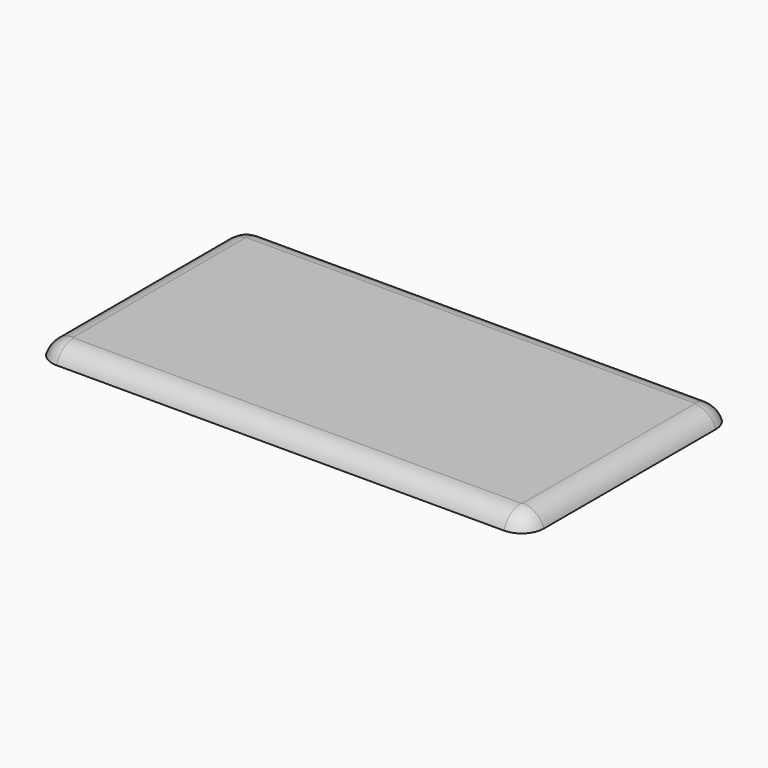
from build123d import *

# Parameters (mm, degrees)
F1_DEPTH     = 3.5
F5_D         = 4.473
F5_DEPTH     = 0.8
F5_TIP       = 1.3438247745
F6_T1_DEPTH  = 101
F6_T3_DEPTH  = 48.5
F6_T6_ANGLE  = 90
F6_T8_ANGLE  = 90
F6_T10_ANGLE = 90
F6_T12_ANGLE = 90
F8_W         = 0.5
F8_H         = 37.5
F8_W_2       = 88
F8_H_2       = 0.5
F9_DEPTH     = 1


# Not quite as in the source:
# - a fillet or chamfer that OpenCascade refuses, or shapes differently, is made with other operations: its cross-section is extruded or revolved along the edge and cut away or added


with BuildPart() as f1:
    # F0 (on Top) → F1 (new body)
    with BuildSketch(Plane.XY):
        with BuildLine():
            Line((-50.5, -29.25), (50.5, -29.25))
            ThreePointArc((50.5, -29.25), (54.0355339059, -27.7855339059), (55.5, -24.25))
            Line((55.5, -24.25), (55.5, 24.25))
            ThreePointArc((55.5, 24.25), (54.0355339059, 27.7855339059), (50.5, 29.25))
            Line((50.5, 29.25), (-50.5, 29.25))
            ThreePointArc((-50.5, 29.25), (-54.0355339059, 27.7855339059), (-55.5, 24.25))
            Line((-55.5, 24.25), (-55.5, -24.25))
            ThreePointArc((-55.5, -24.25), (-54.0355339059, -27.7855339059), (-50.5, -29.25))
        make_face()
    extrude(amount=F1_DEPTH)

    # F5
    with Locations(Plane(origin=(0, 0, 0), x_dir=(1, 0, 0), z_dir=(0, 0, -1))):
        with Locations((-50.2406740561, -23.9985361695), (-50.2495961264, 24.0030474961), (50.2488752827, 23.995583877), (50.2413948998, -24.0000952035)):
            Hole(F5_D / 2, depth=F5_DEPTH)
            with Locations((0, 0, -(F5_DEPTH + F5_TIP / 2))):  # 118° drill point
                Cone(0, F5_D / 2, F5_TIP, mode=Mode.SUBTRACT)

    # F6: fillet of radius 5 on 1 edges, made by hand

    # F6_s2 → F6_t1 (cut)
    with BuildSketch(Plane.YZ.offset(-50.5)):
        with BuildLine():
            ThreePointArc((-29.25, 0), (-27.4383438845, 2.5311288741), (-24.4803039929, 3.5))
            Line((-24.4803039929, 3.5), (-29.25, 3.5))
            Line((-29.25, 3.5), (-29.25, 0))
        make_face()
        with BuildLine():
            ThreePointArc((24.4803039929, 3.5), (27.4383438845, 2.5311288741), (29.25, 0))
            Line((29.25, 0), (29.25, 3.5))
            Line((29.25, 3.5), (24.4803039929, 3.5))
        make_face()
    extrude(amount=F6_T1_DEPTH, mode=Mode.SUBTRACT)

    # F6_s4 → F6_t3 (cut)
    with BuildSketch(Plane.XZ.offset(-24.25)):
        with BuildLine():
            ThreePointArc((50.7303039929, 3.5), (53.6883438845, 2.5311288741), (55.5, 0))
            Line((55.5, 0), (55.5, 3.5))
            Line((55.5, 3.5), (50.7303039929, 3.5))
        make_face()
        with BuildLine():
            ThreePointArc((-50.7303039929, 3.5), (-53.6883438845, 2.5311288741), (-55.5, 0))
            Line((-55.5, 0), (-55.5, 3.5))
            Line((-55.5, 3.5), (-50.7303039929, 3.5))
        make_face()
    extrude(amount=F6_T3_DEPTH, mode=Mode.SUBTRACT)

    # F6_s5 → F6_t6 (revolve, cut)
    with BuildSketch(Plane.XZ.offset(24.25)):
        with BuildLine():
            ThreePointArc((-55.5, 0), (-53.6883438845, 2.5311288741), (-50.7303039929, 3.5))
            Line((-50.7303039929, 3.5), (-55.5, 3.5))
            Line((-55.5, 3.5), (-55.5, 0))
        make_face()
    revolve(axis=Axis((-50.5, -24.25, 3.5), (0, 0, 1)), revolution_arc=F6_T6_ANGLE, mode=Mode.SUBTRACT)

    # F6_s7 → F6_t8 (revolve, cut)
    with BuildSketch(Plane.YZ.offset(50.5)):
        with BuildLine():
            ThreePointArc((-29.25, 0), (-27.4383438845, 2.5311288741), (-24.4803039929, 3.5))
            Line((-24.4803039929, 3.5), (-29.25, 3.5))
            Line((-29.25, 3.5), (-29.25, 0))
        make_face()
    revolve(axis=Axis((50.5, -24.25, 3.5), (0, 0, 1)), revolution_arc=F6_T8_ANGLE, mode=Mode.SUBTRACT)

    # F6_s9 → F6_t10 (revolve, cut)
    with BuildSketch(Plane.XZ.offset(-24.25)):
        with BuildLine():
            ThreePointArc((50.7303039929, 3.5), (53.6883438845, 2.5311288741), (55.5, 0))
            Line((55.5, 0), (55.5, 3.5))
            Line((55.5, 3.5), (50.7303039929, 3.5))
        make_face()
    revolve(axis=Axis((50.5, 24.25, 3.5), (0, 0, 1)), revolution_arc=F6_T10_ANGLE, mode=Mode.SUBTRACT)

    # F6_s11 → F6_t12 (revolve, cut)
    with BuildSketch(Plane.YZ.offset(-50.5)):
        with BuildLine():
            ThreePointArc((24.4803039929, 3.5), (27.4383438845, 2.5311288741), (29.25, 0))
            Line((29.25, 0), (29.25, 3.5))
            Line((29.25, 3.5), (24.4803039929, 3.5))
        make_face()
    revolve(axis=Axis((-50.5, 24.25, 3.5), (0, 0, 1)), revolution_arc=F6_T12_ANGLE, mode=Mode.SUBTRACT)

    # F8 (on Top) → F9 (join)
    with BuildSketch(Plane.XY):
        with Locations((-52.7812354267, 0)):
            Rectangle(F8_W, F8_H)
        with Locations((-0.0016481951, -26.7570052035)):
            Rectangle(F8_W_2, F8_H_2)
        with Locations((52.8098009527, 0)):
            Rectangle(F8_W, F8_H)
        with Locations((-0.0016481951, 26.78494009)):
            Rectangle(F8_W_2, F8_H_2)
    extrude(amount=-F9_DEPTH)


solid = f1.part
